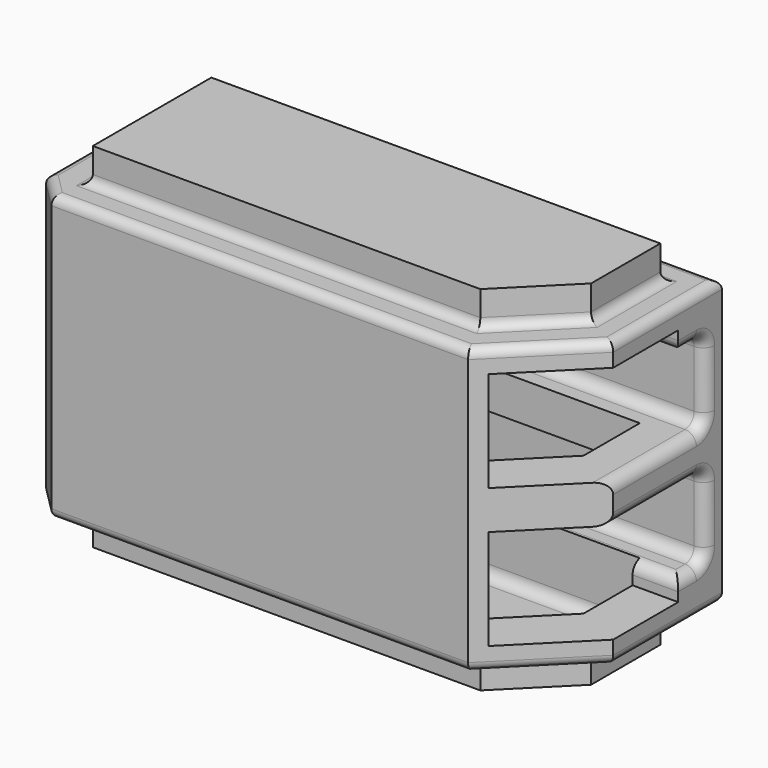
from build123d import *

# Parameters (mm, degrees)
F1_DEPTH = 155
F2_START = 15
F2_DEPTH = 125
F3_R     = 4
F4_W     = 30.3553390593
F4_H     = 44
F5_DEPTH = 215
F4_W_2   = 15
F4_H_2   = 35
F6_DEPTH = 180
F7_START = 5
F7_DEPTH = 145
F8_R     = 5


with BuildPart() as f1:
    # F0 (on Top) → F1 (new body)
    with BuildSketch(Plane.XY):
        Polygon((73, -25), (100, 2), (100, 40), (-97, 40), (-97, -25), align=None)
        Polygon((95, 35), (95, 4.0710678119), (70.9289321881, -20), (-92, -20), (-92, 35), align=None, mode=Mode.SUBTRACT)
        Polygon((70.9289321881, -20), (95, 4.0710678119), (95, 35), (-92, 35), (-92, -20), align=None)
    extrude(amount=F1_DEPTH)

    # F0 (on Top) → F2 (join)
    with BuildSketch(Plane.XY.offset(F2_START)):
        Polygon((-114.6776695297, -28.5355339059), (-103.2132034356, -40), (79.6446609407, -40), (115, -4.6446609407), (115, 55), (-97, 55), (-114.6776695297, 37.3223304703), align=None)
        Polygon((100, 40), (100, 2), (73, -25), (-97, -25), (-97, 40), align=None, mode=Mode.SUBTRACT)
    extrude(amount=F2_DEPTH)

    # F3
    f3_edges = [f1.edges().sort_by_distance(p)[0] for p in [
        (97.32233, -22.32233, 140),
        (115, 25.17767, 140),
        (9, 55, 140),
        (-105.838835, 46.161165, 140),
        (-114.67767, 4.393398, 140),
        (-108.945436, -34.267767, 140),
        (-11.784271, -40, 140),
        (100, 21, 140),
        (86.5, -11.5, 140),
        (-12, -25, 140),
        (-97, 7.5, 140),
        (1.5, 40, 140),
        (97.32233, -22.32233, 15),
        (115, 25.17767, 15),
        (9, 55, 15),
        (-105.838835, 46.161165, 15),
        (-114.67767, 4.393398, 15),
        (-108.945436, -34.267767, 15),
        (-11.784271, -40, 15),
        (100, 21, 15),
        (86.5, -11.5, 15),
        (-12, -25, 15),
        (-97, 7.5, 15),
        (1.5, 40, 15),
    ]]
    fillet(f3_edges, radius=F3_R)

    # F4 (on face) → F5 (cut)
    with BuildSketch(Plane.YZ.offset(115)):
        Polygon((31, 121), (31, 130), (-4.6446609407, 130), (-4.6446609407, 86), (31, 86), align=None)
        with Locations((-19.8223304703, 108)):
            Rectangle(F4_W, F4_H)
        with Locations((-19.8223304703, 47)):
            Rectangle(F4_W, F4_H)
        Polygon((31, 69), (-4.6446609407, 69), (-4.6446609407, 25), (31, 25), (31, 34), align=None)
    extrude(amount=-F5_DEPTH, mode=Mode.SUBTRACT)

    # F4 (on face) → F6 (cut)
    with BuildSketch(Plane.YZ.offset(115)):
        with Locations((38.5, 51.5)):
            Rectangle(F4_W_2, F4_H_2)
        with Locations((38.5, 103.5)):
            Rectangle(F4_W_2, F4_H_2)
    extrude(amount=-F6_DEPTH, mode=Mode.SUBTRACT)

    # F0 (on Top) → F7 (cut)
    with BuildSketch(Plane.XY.offset(F7_START)):
        Polygon((70.9289321881, -20), (95, 4.0710678119), (95, 35), (-92, 35), (-92, -20), align=None)
    extrude(amount=F7_DEPTH, mode=Mode.SUBTRACT)

    # F8
    f8_edges = [f1.edges().sort_by_distance(p)[0] for p in [
        (105, 31, 121),
        (105, 31, 34),
        (-100, 31, 108),
        (-100, -2, 130),
        (-100, -35, 108),
        (-100, -2, 86),
        (-100, -35, 47),
        (-100, -2, 25),
        (-100, 31, 47),
        (-100, -2, 69),
        (82.964466, -7.964466, 5),
        (95, 19.535534, 5),
        (1.5, 35, 5),
        (-92, 7.5, 5),
        (-10.535534, -20, 5),
        (82.964466, -7.964466, 150),
        (95, 19.535534, 150),
        (1.5, 35, 150),
        (-92, 7.5, 150),
        (-10.535534, -20, 150),
        (25, 46, 86),
        (25, 46, 121),
        (115, 46, 103.5),
        (-65, 46, 103.5),
        (25, 46, 34),
        (25, 46, 69),
        (115, 46, 51.5),
        (-65, 46, 51.5),
        (115, 38.5, 34),
        (115, 20.67767, 69),
        (115, 20.67767, 86),
        (115, 38.5, 121),
    ]]
    fillet(f8_edges, radius=F8_R)


solid = f1.part
